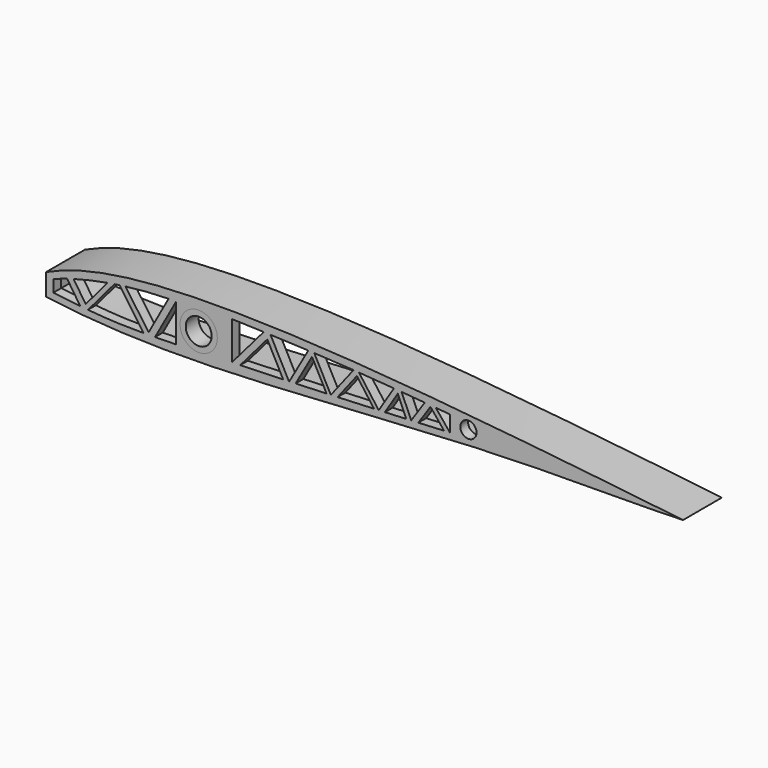
from build123d import *

# Parameters (mm, degrees)
F0_R     = 5.75
F0_R_2   = 2.5
F1_DEPTH = 3
F2_DEPTH = 15
F0_R_3   = 4
F3_DEPTH = 5


# Not quite as in the source:
# - ends of sketch curves that miss each other by under 0.0002 mm in the source are joined


with BuildPart() as f1:
    # F0 (on Front) → F1 (new body)
    with BuildSketch(Plane.XZ):
        with BuildLine():
            add(Edge.make_bspline(
                [(-96.5428803444, -1.7252441192), (-96.4749771743, -1.6951094214), (-96.406839482, -1.6654244391), (-96.3385477662, -1.6362179573)],
                knots=[0.9799990925, 0.9799990925, 0.9799990925, 0.9799990925, 1, 1, 1, 1], degree=3))
            Line((-96.5428803444, -1.7252441192), (-96.5428803444, -6.1999121678))
            add(Edge.make_bspline(
                [(-96.5428803445, -6.1999121678), (-96.1611087474, -6.2678718719), (-95.7782117135, -6.3340115071), (-95.3941463942, -6.3983665862)],
                knots=[0.0058166358, 0.0058166358, 0.0058166358, 0.0058166358, 0.0137332718, 0.0137332718, 0.0137332718, 0.0137332718], degree=3))
            Line((-95.3941463942, -6.3983665862), (-95.3941463942, -1.2117682704))
            add(Edge.make_bspline(
                [(-96.3385477662, -1.6362179573), (-96.0300606253, -1.4927727074), (-95.71523374, -1.3512900387), (-95.3941463942, -1.2117682704)],
                knots=[0, 0, 0, 0, 0.0112083174, 0.0112083174, 0.0112083174, 0.0112083174], degree=3))
        make_face()
        with BuildLine():
            Line((-95.3941463942, -1.2117682704), (-95.3941463942, -6.3983665862))
            add(Edge.make_bspline(
                [(-95.3941463942, -6.3983665862), (-80.8694306992, -8.8321693274), (-43.0853796331, -8.5556683111), (40.9195716837, -3.3120714751), (72.7341022162, -3.1550192186), (86.094097513, -3.3751911245)],
                knots=[0.0137332718, 0.0137332718, 0.0137332718, 0.0137332718, 0.3131273629, 0.7122131732, 1, 1, 1, 1], degree=3))
            add(Edge.make_bspline(
                [(-95.3941463942, -1.2117682704), (-84.6882492469, 3.4402546795), (-37.9471480513, 9.9808619504), (36.943279708, 1.696590452), (86.094097513, -3.3751911245)],
                knots=[0.0112083174, 0.0112083174, 0.0112083174, 0.0112083174, 0.384923117, 1, 1, 1, 1], degree=3))
        make_face()
        with BuildLine():
            add(Edge.make_bspline(
                [(-58.7596564737, 4.4301702308), (-57.9753522042, 4.4434334419), (-57.1958768535, 4.4485089516), (-56.4223485914, 4.4453240584)],
                knots=[0.9373807911, 0.9373807911, 0.9373807911, 0.9373807911, 1, 1, 1, 1], degree=3))
            Line((-56.4223485914, 4.4453240584), (-56.4223485914, -7.2081234653))
            add(Edge.make_bspline(
                [(-56.4223485914, -7.2081234653), (-58.5959136423, -7.2589059214), (-60.7694786933, -7.3096883775), (-62.937808184, -7.3435649348)],
                knots=[0, 0, 0, 0, 0.1686137564, 0.1686137564, 0.1686137564, 0.1686137564], degree=3))
            add(Edge.make_bspline(
                [(-62.937808184, -7.3435649348), (-64.1162804896, -7.3619766129), (-65.2932062899, -7.3753945447), (-66.4677450702, -7.3811046631)],
                knots=[0.1686137564, 0.1686137564, 0.1686137564, 0.1686137564, 0.2602541842, 0.2602541842, 0.2602541842, 0.2602541842], degree=3))
            add(Edge.make_bspline(
                [(-66.4677450702, -7.3811046631), (-69.6195281104, -7.3964273197), (-75.381287574, -7.3225727781), (-81.0300999392, -6.8840061254), (-83.592082751, -6.6398550354)],
                knots=[0.2602541842, 0.2602541842, 0.2602541842, 0.2602541842, 0.5061641117, 0.7122660034, 0.7122660034, 0.7122660034, 0.7122660034], degree=3))
            add(Edge.make_bspline(
                [(-83.592082751, -6.6398550354), (-84.4022359708, -6.5626492904), (-85.2110210526, -6.4810257561), (-86.0187478894, -6.3959850932)],
                knots=[0.7122660034, 0.7122660034, 0.7122660034, 0.7122660034, 0.7774397861, 0.7774397861, 0.7774397861, 0.7774397861], degree=3))
            add(Edge.make_bspline(
                [(-86.0187478894, -6.3959850932), (-88.7770327399, -6.1055819993), (-91.5229770142, -5.7753305369), (-94.2689212885, -5.4450790744)],
                knots=[0.7774397861, 0.7774397861, 0.7774397861, 0.7774397861, 1, 1, 1, 1], degree=3))
            Line((-94.2689212885, -5.4450790744), (-94.2689212885, -1.6795024276))
            add(Edge.make_bspline(
                [(-94.2689212885, -1.6795024276), (-92.8628953972, -1.1841994891), (-91.4581917851, -0.7250541475), (-90.0523380192, -0.2995832154)],
                knots=[0, 0, 0, 0, 0.113305349, 0.113305349, 0.113305349, 0.113305349], degree=3))
            add(Edge.make_bspline(
                [(-90.0523380192, -0.2995832154), (-89.3811327558, -0.0964480559), (-88.7096653203, 0.0990111844), (-88.0376666398, 0.2870647488)],
                knots=[0.113305349, 0.113305349, 0.113305349, 0.113305349, 0.1674014069, 0.1674014069, 0.1674014069, 0.1674014069], degree=3))
            add(Edge.make_bspline(
                [(-88.0376666398, 0.2870647488), (-84.5719605974, 1.2569154246), (-81.0921245769, 2.0297910107), (-77.561248917, 2.6427617143)],
                knots=[0.1674014069, 0.1674014069, 0.1674014069, 0.1674014069, 0.4463915894, 0.4463915894, 0.4463915894, 0.4463915894], degree=3))
            add(Edge.make_bspline(
                [(-77.561248917, 2.6427617143), (-76.8555880554, 2.7652665761), (-76.1478885806, 2.8813845552), (-75.4378558602, 2.991411566)],
                knots=[0.4463915894, 0.4463915894, 0.4463915894, 0.4463915894, 0.5021489911, 0.5021489911, 0.5021489911, 0.5021489911], degree=3))
            add(Edge.make_bspline(
                [(-75.4378558602, 2.991411566), (-74.9289069597, 3.0702785315), (-74.4187592444, 3.1460159753), (-73.9077034377, 3.2186049948)],
                knots=[0.5021489911, 0.5021489911, 0.5021489911, 0.5021489911, 0.5421156961, 0.5421156961, 0.5421156961, 0.5421156961], degree=3))
            add(Edge.make_bspline(
                [(-73.9077034377, 3.2186049948), (-73.2834974958, 3.3072655612), (-72.6579368364, 3.3912292161), (-72.0315511948, 3.4704615167)],
                knots=[0.5421156961, 0.5421156961, 0.5421156961, 0.5421156961, 0.5909312157, 0.5909312157, 0.5909312157, 0.5909312157], degree=3))
            add(Edge.make_bspline(
                [(-72.0315511948, 3.4704615167), (-67.5860174529, 4.0327826216), (-63.0989300921, 4.3567896513), (-58.7596564737, 4.4301702308)],
                knots=[0.5909312157, 0.5909312157, 0.5909312157, 0.5909312157, 0.9373807911, 0.9373807911, 0.9373807911, 0.9373807911], degree=3))
        make_face(mode=Mode.SUBTRACT)
        with Locations((-49.452, -1.371)):
            Circle(F0_R, mode=Mode.SUBTRACT)
        with BuildLine():
            Line((-39.2314642668, -6.5102223307), (-39.2314642668, 5.299675744))
            add(Edge.make_bspline(
                [(-39.2314642668, 5.299675744), (-35.9534074438, 5.1909875249), (-32.6753506208, 5.0822993057), (-29.3931825657, 4.965637255)],
                knots=[0, 0, 0, 0, 0.1482033118, 0.1482033118, 0.1482033118, 0.1482033118], degree=3))
            add(Edge.make_bspline(
                [(-29.3931825657, 4.965637255), (-28.6917369238, 4.940704928), (-27.9901035066, 4.9154084065), (-27.2882421839, 4.8896698568)],
                knots=[0.1482033118, 0.1482033118, 0.1482033118, 0.1482033118, 0.1798764515, 0.1798764515, 0.1798764515, 0.1798764515], degree=3))
            add(Edge.make_bspline(
                [(-27.2882421839, 4.8896698568), (-23.4137483209, 4.7475850185), (-19.5323092994, 4.5920298819), (-15.6371742048, 4.4099108889)],
                knots=[0.1798764515, 0.1798764515, 0.1798764515, 0.1798764515, 0.3547220816, 0.3547220816, 0.3547220816, 0.3547220816], degree=3))
            add(Edge.make_bspline(
                [(-15.6371742048, 4.4099108889), (-15.0215280405, 4.3811260441), (-14.4055397287, 4.3516775961), (-13.7891826138, 4.3215138457)],
                knots=[0.3547220816, 0.3547220816, 0.3547220816, 0.3547220816, 0.382357334, 0.382357334, 0.382357334, 0.382357334], degree=3))
            add(Edge.make_bspline(
                [(-13.7891826138, 4.3215138457), (-11.2804707946, 4.1987406107), (-7.2510801006, 3.9830392372), (-3.2013896807, 3.7279660672), (-1.676706941, 3.6272723386)],
                knots=[0.382357334, 0.382357334, 0.382357334, 0.382357334, 0.4948390149, 0.5625818971, 0.5625818971, 0.5625818971, 0.5625818971], degree=3))
            add(Edge.make_bspline(
                [(-1.676706941, 3.6272723386), (-1.1181316432, 3.5903826775), (-0.5592230256, 3.552846535), (0, 3.5147005908)],
                knots=[0.5625818971, 0.5625818971, 0.5625818971, 0.5625818971, 0.5873998474, 0.5873998474, 0.5873998474, 0.5873998474], degree=3))
            add(Edge.make_bspline(
                [(0, 3.5147005908), (3.5849822281, 3.2701603521), (7.1828854983, 3.000559448), (10.7887274401, 2.7155613037)],
                knots=[0.5873998474, 0.5873998474, 0.5873998474, 0.5873998474, 0.7464990028, 0.7464990028, 0.7464990028, 0.7464990028], degree=3))
            add(Edge.make_bspline(
                [(10.7887274401, 2.7155613037), (11.5803406425, 2.6529938652), (12.3723364586, 2.5896843385), (13.1646621709, 2.5257349704)],
                knots=[0.7464990028, 0.7464990028, 0.7464990028, 0.7464990028, 0.7814270428, 0.7814270428, 0.7814270428, 0.7814270428], degree=3))
            add(Edge.make_bspline(
                [(13.1646621709, 2.5257349704), (15.5409627422, 2.3339414724), (17.9202306891, 2.1363926795), (20.3010438532, 1.9358469013)],
                knots=[0.7814270428, 0.7814270428, 0.7814270428, 0.7814270428, 0.8861813381, 0.8861813381, 0.8861813381, 0.8861813381], degree=3))
            add(Edge.make_bspline(
                [(20.3010438532, 1.9358469013), (21.4384423664, 1.8400391019), (22.5761935461, 1.7435472975), (23.7141423287, 1.6466722377)],
                knots=[0.8861813381, 0.8861813381, 0.8861813381, 0.8861813381, 0.9362261637, 0.9362261637, 0.9362261637, 0.9362261637], degree=3))
            add(Edge.make_bspline(
                [(23.7141423287, 1.6466722377), (25.1642694588, 1.523221029), (26.6147174818, 1.3991474412), (28.0651655048, 1.2750738533)],
                knots=[0.9362261637, 0.9362261637, 0.9362261637, 0.9362261637, 1, 1, 1, 1], degree=3))
            Line((28.0651655048, 1.2750738533), (28.0651655048, -3.6732077133))
            add(Edge.make_bspline(
                [(28.0651655048, -3.6732077133), (27.4664662691, -3.7032045951), (26.8677670333, -3.7332014769), (26.269106513, -3.7631839579)],
                knots=[0, 0, 0, 0, 0.0260461999, 0.0260461999, 0.0260461999, 0.0260461999], degree=3))
            add(Edge.make_bspline(
                [(26.269106513, -3.7631839579), (23.6217461688, -3.8957706721), (20.9751429176, -4.0280757752), (18.3326447297, -4.1588539429)],
                knots=[0.0260461999, 0.0260461999, 0.0260461999, 0.0260461999, 0.1412261299, 0.1412261299, 0.1412261299, 0.1412261299], degree=3))
            add(Edge.make_bspline(
                [(18.3326447297, -4.1588539429), (17.592409558, -4.1954884427), (16.8524965153, -4.2320031222), (16.1129791965, -4.2683706067)],
                knots=[0.1412261299, 0.1412261299, 0.1412261299, 0.1412261299, 0.1734911417, 0.1734911417, 0.1734911417, 0.1734911417], degree=3))
            add(Edge.make_bspline(
                [(16.1129791965, -4.2683706067), (15.6061303016, -4.2932960802), (15.0994672951, -4.3181524099), (14.5930138711, -4.3429307826)],
                knots=[0.1734911417, 0.1734911417, 0.1734911417, 0.1734911417, 0.1956048707, 0.1956048707, 0.1956048707, 0.1956048707], degree=3))
            add(Edge.make_bspline(
                [(14.5930138711, -4.3429307826), (12.3936169659, -4.4505368792), (10.1981726621, -4.5566727509), (8.0086215303, -4.6606165755)],
                knots=[0.1956048707, 0.1956048707, 0.1956048707, 0.1956048707, 0.2916391057, 0.2916391057, 0.2916391057, 0.2916391057], degree=3))
            add(Edge.make_bspline(
                [(8.0086215303, -4.6606165755), (7.3735996711, -4.6907627547), (6.739073509, -4.7207245525), (6.105090384, -4.7504843601)],
                knots=[0.2916391057, 0.2916391057, 0.2916391057, 0.2916391057, 0.3194913159, 0.3194913159, 0.3194913159, 0.3194913159], degree=3))
            add(Edge.make_bspline(
                [(6.105090384, -4.7504843601), (5.6209562477, -4.773210105), (5.1371387803, -4.7958180605), (4.6536590632, -4.818300385)],
                knots=[0.3194913159, 0.3194913159, 0.3194913159, 0.3194913159, 0.3407603453, 0.3407603453, 0.3407603453, 0.3407603453], degree=3))
            add(Edge.make_bspline(
                [(4.6536590632, -4.818300385), (0.8798372036, -4.9937871426), (-2.8734067176, -5.1616196506), (-6.5960472566, -5.3180688061)],
                knots=[0.3407603453, 0.3407603453, 0.3407603453, 0.3407603453, 0.5067766752, 0.5067766752, 0.5067766752, 0.5067766752], degree=3))
            add(Edge.make_bspline(
                [(-6.5960472566, -5.3180688061), (-6.6322875139, -5.3195918534), (-7.325510614, -5.3487072139), (-8.0176689199, -5.3774265095), (-8.6727461513, -5.4043100041)],
                knots=[0.5067766752, 0.5067766752, 0.5067766752, 0.5067766752, 0.5083928599, 0.5376943974, 0.5376943974, 0.5376943974, 0.5376943974], degree=3))
            add(Edge.make_bspline(
                [(-8.6727461513, -5.4043100041), (-9.1152981748, -5.422471748), (-9.557439724, -5.4404808103), (-9.9991883747, -5.4583437286)],
                knots=[0.5376943974, 0.5376943974, 0.5376943974, 0.5376943974, 0.5574897042, 0.5574897042, 0.5574897042, 0.5574897042], degree=3))
            add(Edge.make_bspline(
                [(-9.9991883747, -5.4583437286), (-13.1995651312, -5.5877568424), (-16.3793198272, -5.7094992948), (-19.5451358525, -5.8260570653)],
                knots=[0.5574897042, 0.5574897042, 0.5574897042, 0.5574897042, 0.7009025691, 0.7009025691, 0.7009025691, 0.7009025691], degree=3))
            add(Edge.make_bspline(
                [(-19.5451358525, -5.8260570653), (-20.1920530868, -5.8498750098), (-20.8383882883, -5.8734764592), (-21.4841984848, -5.8968826257)],
                knots=[0.7009025691, 0.7009025691, 0.7009025691, 0.7009025691, 0.7302082057, 0.7302082057, 0.7302082057, 0.7302082057], degree=3))
            add(Edge.make_bspline(
                [(-21.4841984848, -5.8968826257), (-21.5265905055, -5.8984190441), (-21.568980264, -5.8999546211), (-21.6113677766, -5.9014893627)],
                knots=[0.7302082057, 0.7302082057, 0.7302082057, 0.7302082057, 0.7321318749, 0.7321318749, 0.7321318749, 0.7321318749], degree=3))
            add(Edge.make_bspline(
                [(-21.6113677766, -5.9014893627), (-22.2032423382, -5.9229196008), (-22.7946789769, -5.9441869474), (-23.3857216062, -5.9653077367)],
                knots=[0.7321318749, 0.7321318749, 0.7321318749, 0.7321318749, 0.7589928716, 0.7589928716, 0.7589928716, 0.7589928716], degree=3))
            add(Edge.make_bspline(
                [(-23.3857216062, -5.9653077367), (-27.8246304727, -6.1239312512), (-32.2413153798, -6.2742882557), (-36.6543788181, -6.4232982046)],
                knots=[0.7589928716, 0.7589928716, 0.7589928716, 0.7589928716, 0.9607270796, 0.9607270796, 0.9607270796, 0.9607270796], degree=3))
            add(Edge.make_bspline(
                [(-36.6543788181, -6.4232982046), (-37.5134988009, -6.452306948), (-38.3724815339, -6.4812646393), (-39.2314642668, -6.5102223307)],
                knots=[0.9607270796, 0.9607270796, 0.9607270796, 0.9607270796, 1, 1, 1, 1], degree=3))
        make_face(mode=Mode.SUBTRACT)
        with Locations((33.779, -1.031)):
            Circle(F0_R_2, mode=Mode.SUBTRACT)
        with BuildLine():
            Line((-62.937808184, -7.3435649348), (-56.4223485914, 4.4453240584))
            add(Edge.make_bspline(
                [(-58.7596564737, 4.4301702308), (-57.9753522042, 4.4434334419), (-57.1958768535, 4.4485089516), (-56.4223485914, 4.4453240584)],
                knots=[0.9373807911, 0.9373807911, 0.9373807911, 0.9373807911, 1, 1, 1, 1], degree=3))
            Line((-58.7596564737, 4.4301702308), (-64.903050668, -6.6855141148))
            Line((-64.903050668, -6.6855141148), (-72.0315511948, 3.4704615167))
            add(Edge.make_bspline(
                [(-73.9077034377, 3.2186049948), (-73.2834974958, 3.3072655612), (-72.6579368364, 3.3912292161), (-72.0315511948, 3.4704615167)],
                knots=[0.5421156961, 0.5421156961, 0.5421156961, 0.5421156961, 0.5909312157, 0.5909312157, 0.5909312157, 0.5909312157], degree=3))
            Line((-73.9077034377, 3.2186049948), (-66.4677450702, -7.3811046631))
            add(Edge.make_bspline(
                [(-62.937808184, -7.3435649348), (-64.1162804896, -7.3619766129), (-65.2932062899, -7.3753945447), (-66.4677450702, -7.3811046631)],
                knots=[0.1686137564, 0.1686137564, 0.1686137564, 0.1686137564, 0.2602541842, 0.2602541842, 0.2602541842, 0.2602541842], degree=3))
        make_face()
        with BuildLine():
            add(Edge.make_bspline(
                [(-83.592082751, -6.6398550354), (-84.4022359708, -6.5626492904), (-85.2110210526, -6.4810257561), (-86.0187478894, -6.3959850932)],
                knots=[0.7122660034, 0.7122660034, 0.7122660034, 0.7122660034, 0.7774397861, 0.7774397861, 0.7774397861, 0.7774397861], degree=3))
            Line((-83.592082751, -6.6398550354), (-75.4378558602, 2.991411566))
            add(Edge.make_bspline(
                [(-77.561248917, 2.6427617143), (-76.8555880554, 2.7652665761), (-76.1478885806, 2.8813845552), (-75.4378558602, 2.991411566)],
                knots=[0.4463915894, 0.4463915894, 0.4463915894, 0.4463915894, 0.5021489911, 0.5021489911, 0.5021489911, 0.5021489911], degree=3))
            Line((-77.561248917, 2.6427617143), (-84.3168773909, -5.3365672599))
            Line((-84.3168773909, -5.3365672599), (-88.0376666398, 0.2870647488))
            add(Edge.make_bspline(
                [(-90.0523380192, -0.2995832154), (-89.3811327558, -0.0964480559), (-88.7096653203, 0.0990111844), (-88.0376666398, 0.2870647488)],
                knots=[0.113305349, 0.113305349, 0.113305349, 0.113305349, 0.1674014069, 0.1674014069, 0.1674014069, 0.1674014069], degree=3))
            Line((-90.0523380192, -0.2995832154), (-86.0187478894, -6.3959850932))
        make_face()
        with BuildLine():
            Line((-29.3931825657, 4.965637255), (-39.2314642668, -6.5102223307))
            add(Edge.make_bspline(
                [(-36.6543788181, -6.4232982046), (-37.5134988009, -6.452306948), (-38.3724815339, -6.4812646393), (-39.2314642668, -6.5102223307)],
                knots=[0.9607270796, 0.9607270796, 0.9607270796, 0.9607270796, 1, 1, 1, 1], degree=3))
            Line((-36.6543788181, -6.4232982046), (-28.2822091366, 3.3424156275))
            Line((-28.2822091366, 3.3424156275), (-23.3857216062, -5.9653077367))
            add(Edge.make_bspline(
                [(-21.6113677766, -5.9014893627), (-22.2032423382, -5.9229196008), (-22.7946789769, -5.9441869474), (-23.3857216062, -5.9653077367)],
                knots=[0.7321318749, 0.7321318749, 0.7321318749, 0.7321318749, 0.7589928716, 0.7589928716, 0.7589928716, 0.7589928716], degree=3))
            Line((-21.6113677766, -5.9014893627), (-27.2882421839, 4.8896698568))
            add(Edge.make_bspline(
                [(-29.3931825657, 4.965637255), (-28.6917369238, 4.940704928), (-27.9901035066, 4.9154084065), (-27.2882421839, 4.8896698568)],
                knots=[0.1482033118, 0.1482033118, 0.1482033118, 0.1482033118, 0.1798764515, 0.1798764515, 0.1798764515, 0.1798764515], degree=3))
        make_face()
        with BuildLine():
            add(Edge.make_bspline(
                [(-15.6371742048, 4.4099108889), (-15.0215280405, 4.3811260441), (-14.4055397287, 4.3516775961), (-13.7891826138, 4.3215138457)],
                knots=[0.3547220816, 0.3547220816, 0.3547220816, 0.3547220816, 0.382357334, 0.382357334, 0.382357334, 0.382357334], degree=3))
            Line((-15.6371742048, 4.4099108889), (-21.4841984848, -5.8968826257))
            add(Edge.make_bspline(
                [(-19.5451358525, -5.8260570653), (-20.1920530868, -5.8498750098), (-20.8383882883, -5.8734764592), (-21.4841984848, -5.8968826257)],
                knots=[0.7009025691, 0.7009025691, 0.7009025691, 0.7009025691, 0.7302082057, 0.7302082057, 0.7302082057, 0.7302082057], degree=3))
            Line((-19.5451358525, -5.8260570653), (-14.4918043747, 3.0816610505))
            Line((-14.4918043747, 3.0816610505), (-9.9991883747, -5.4583437286))
            add(Edge.make_bspline(
                [(-8.6727461513, -5.4043100041), (-9.1152981748, -5.422471748), (-9.557439724, -5.4404808103), (-9.9991883747, -5.4583437286)],
                knots=[0.5376943974, 0.5376943974, 0.5376943974, 0.5376943974, 0.5574897042, 0.5574897042, 0.5574897042, 0.5574897042], degree=3))
            Line((-8.6727461513, -5.4043100041), (-13.7891826138, 4.3215138457))
        make_face()
        with BuildLine():
            add(Edge.make_bspline(
                [(-1.676706941, 3.6272723386), (-1.1181316432, 3.5903826775), (-0.5592230256, 3.552846535), (0, 3.5147005908)],
                knots=[0.5625818971, 0.5625818971, 0.5625818971, 0.5625818971, 0.5873998474, 0.5873998474, 0.5873998474, 0.5873998474], degree=3))
            Line((-1.676706941, 3.6272723386), (-8.6727461513, -5.4043100041))
            add(Edge.make_bspline(
                [(-6.5960472566, -5.3180688061), (-6.6322875139, -5.3195918534), (-7.325510614, -5.3487072139), (-8.0176689199, -5.3774265095), (-8.6727461513, -5.4043100041)],
                knots=[0.5067766752, 0.5067766752, 0.5067766752, 0.5067766752, 0.5083928599, 0.5376943974, 0.5376943974, 0.5376943974, 0.5376943974], degree=3))
            Line((-6.5960472566, -5.3180688061), (-0.6485358524, 2.3599097423))
            Line((-0.6485358524, 2.3599097423), (4.6536590632, -4.818300385))
            add(Edge.make_bspline(
                [(6.105090384, -4.7504843601), (5.6209562477, -4.773210105), (5.1371387803, -4.7958180605), (4.6536590632, -4.818300385)],
                knots=[0.3194913159, 0.3194913159, 0.3194913159, 0.3194913159, 0.3407603453, 0.3407603453, 0.3407603453, 0.3407603453], degree=3))
            Line((6.105090384, -4.7504843601), (0, 3.5147005908))
        make_face()
        with BuildLine():
            add(Edge.make_bspline(
                [(10.7887274401, 2.7155613037), (11.5803406425, 2.6529938652), (12.3723364586, 2.5896843385), (13.1646621709, 2.5257349704)],
                knots=[0.7464990028, 0.7464990028, 0.7464990028, 0.7464990028, 0.7814270428, 0.7814270428, 0.7814270428, 0.7814270428], degree=3))
            Line((10.7887274401, 2.7155613037), (6.105090384, -4.7504843601))
            add(Edge.make_bspline(
                [(8.0086215303, -4.6606165755), (7.3735996711, -4.6907627547), (6.739073509, -4.7207245525), (6.105090384, -4.7504843601)],
                knots=[0.2916391057, 0.2916391057, 0.2916391057, 0.2916391057, 0.3194913159, 0.3194913159, 0.3194913159, 0.3194913159], degree=3))
            Line((8.0086215303, -4.6606165755), (11.9821707942, 1.6734993897))
            Line((11.9821707942, 1.6734993897), (14.5930138711, -4.3429307826))
            add(Edge.make_bspline(
                [(16.1129791965, -4.2683706067), (15.6061303016, -4.2932960802), (15.0994672951, -4.3181524099), (14.5930138711, -4.3429307826)],
                knots=[0.1734911417, 0.1734911417, 0.1734911417, 0.1734911417, 0.1956048707, 0.1956048707, 0.1956048707, 0.1956048707], degree=3))
            Line((16.1129791965, -4.2683706067), (13.1646621709, 2.5257349704))
        make_face()
        with BuildLine():
            add(Edge.make_bspline(
                [(20.3010438532, 1.9358469013), (21.4384423664, 1.8400391019), (22.5761935461, 1.7435472975), (23.7141423287, 1.6466722377)],
                knots=[0.8861813381, 0.8861813381, 0.8861813381, 0.8861813381, 0.9362261637, 0.9362261637, 0.9362261637, 0.9362261637], degree=3))
            Line((20.3010438532, 1.9358469013), (16.1129791965, -4.2683706067))
            add(Edge.make_bspline(
                [(18.3326447297, -4.1588539429), (17.592409558, -4.1954884427), (16.8524965153, -4.2320031222), (16.1129791965, -4.2683706067)],
                knots=[0.1412261299, 0.1412261299, 0.1412261299, 0.1412261299, 0.1734911417, 0.1734911417, 0.1734911417, 0.1734911417], degree=3))
            Line((18.3326447297, -4.1588539429), (22.0675114827, 1.3739941859))
            Line((22.0675114827, 1.3739941859), (26.269106513, -3.7631839579))
            add(Edge.make_bspline(
                [(28.0651655048, -3.6732077133), (27.4664662691, -3.7032045951), (26.8677670333, -3.7332014769), (26.269106513, -3.7631839579)],
                knots=[0, 0, 0, 0, 0.0260461999, 0.0260461999, 0.0260461999, 0.0260461999], degree=3))
            Line((28.0651655048, -3.6732077133), (23.7141423287, 1.6466722377))
        make_face()
    extrude(amount=-F1_DEPTH)

    # F0 (on Front) → F2 (join)
    with BuildSketch(Plane.XZ):
        with BuildLine():
            add(Edge.make_bspline(
                [(-96.5428803444, -0.598909816), (-84.374379176, 5.1984880484), (-38.2751930486, 10.925719155), (42.6881882799, 2.4723259958), (100, -4.047003109)],
                knots=[0.0044628662, 0.0044628662, 0.0044628662, 0.0044628662, 0.374886421, 1, 1, 1, 1], degree=3))
            Line((-96.5428803444, -0.598909816), (-96.5428803444, -1.7252441192))
            add(Edge.make_bspline(
                [(-96.5428803444, -1.7252441192), (-96.4749771743, -1.6951094214), (-96.406839482, -1.6654244391), (-96.3385477662, -1.6362179573)],
                knots=[0.9799990925, 0.9799990925, 0.9799990925, 0.9799990925, 1, 1, 1, 1], degree=3))
            add(Edge.make_bspline(
                [(-96.3385477662, -1.6362179573), (-96.0300606253, -1.4927727074), (-95.71523374, -1.3512900387), (-95.3941463942, -1.2117682704)],
                knots=[0, 0, 0, 0, 0.0112083174, 0.0112083174, 0.0112083174, 0.0112083174], degree=3))
            add(Edge.make_bspline(
                [(-95.3941463942, -1.2117682704), (-84.6882492469, 3.4402546795), (-37.9471480513, 9.9808619504), (36.943279708, 1.696590452), (86.094097513, -3.3751911245)],
                knots=[0.0112083174, 0.0112083174, 0.0112083174, 0.0112083174, 0.384923117, 1, 1, 1, 1], degree=3))
            add(Edge.make_bspline(
                [(-95.3941463942, -6.3983665862), (-80.8694306992, -8.8321693274), (-43.0853796331, -8.5556683111), (40.9195716837, -3.3120714751), (72.7341022162, -3.1550192186), (86.094097513, -3.3751911245)],
                knots=[0.0137332718, 0.0137332718, 0.0137332718, 0.0137332718, 0.3131273629, 0.7122131732, 1, 1, 1, 1], degree=3))
            add(Edge.make_bspline(
                [(-96.5428803445, -6.1999121678), (-96.1611087474, -6.2678718719), (-95.7782117135, -6.3340115071), (-95.3941463942, -6.3983665862)],
                knots=[0.0058166358, 0.0058166358, 0.0058166358, 0.0058166358, 0.0137332718, 0.0137332718, 0.0137332718, 0.0137332718], degree=3))
            Line((-96.5428803445, -6.1999121678), (-96.5428803444, -7.3406707446))
            add(Edge.make_bspline(
                [(-96.5428803444, -7.3406707446), (-80.7020161693, -9.4302402111), (-44.2471235075, -11.1181020976), (41.8622965332, -3.5518856086), (82.0915186506, -4.6802794425), (100, -4.047003109)],
                knots=[0, 0, 0, 0, 0.2987594418, 0.6837410955, 1, 1, 1, 1], degree=3))
        make_face()
        with BuildLine():
            add(Edge.make_bspline(
                [(-96.5428803444, -1.7252441192), (-96.4749771743, -1.6951094214), (-96.406839482, -1.6654244391), (-96.3385477662, -1.6362179573)],
                knots=[0.9799990925, 0.9799990925, 0.9799990925, 0.9799990925, 1, 1, 1, 1], degree=3))
            Line((-96.5428803444, -1.7252441192), (-96.5428803444, -6.1999121678))
            add(Edge.make_bspline(
                [(-96.5428803445, -6.1999121678), (-96.1611087474, -6.2678718719), (-95.7782117135, -6.3340115071), (-95.3941463942, -6.3983665862)],
                knots=[0.0058166358, 0.0058166358, 0.0058166358, 0.0058166358, 0.0137332718, 0.0137332718, 0.0137332718, 0.0137332718], degree=3))
            Line((-95.3941463942, -6.3983665862), (-95.3941463942, -1.2117682704))
            add(Edge.make_bspline(
                [(-96.3385477662, -1.6362179573), (-96.0300606253, -1.4927727074), (-95.71523374, -1.3512900387), (-95.3941463942, -1.2117682704)],
                knots=[0, 0, 0, 0, 0.0112083174, 0.0112083174, 0.0112083174, 0.0112083174], degree=3))
        make_face()
    extrude(amount=-F2_DEPTH)


with BuildPart() as f3:
    # F0 (on Front) → F3 (new body)
    with BuildSketch(Plane.XZ):
        with Locations((-49.452, -1.371)):
            Circle(F0_R)
        with Locations((-49.452, -1.371)):
            Circle(F0_R_3, mode=Mode.SUBTRACT)
    extrude(amount=-F3_DEPTH)


solid = Compound([f1.part, f3.part])
